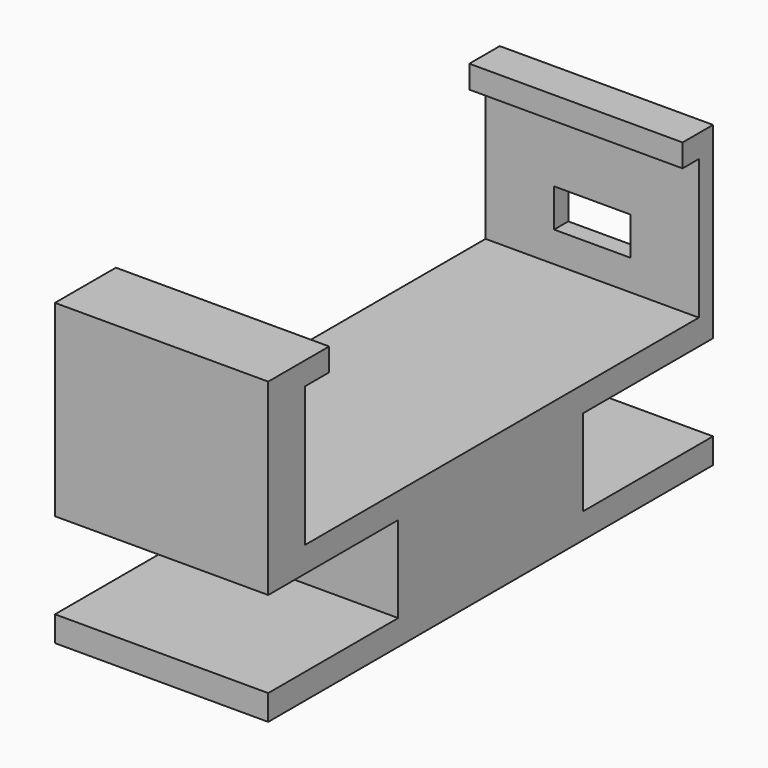
from build123d import *

# Parameters (mm, degrees)
F0_W      = 42
F0_H      = 109.5
F1_DEPTH  = 5
F2_W      = 42
F2_H      = 7.5
F2_H_2    = 15
F3_DEPTH  = 32
F4_W      = 42
F4_H      = 27.5
F5_DEPTH  = 4
F6_W      = 42
F6_H      = 27.5
F7_DEPTH  = 6
F8_W      = 15
F8_H      = 7.5
F9_DEPTH  = 3.501
F10_W     = 42
F10_H     = 54.75
F11_DEPTH = 22
F12_W     = 42
F12_H     = 17
F13_DEPTH = 32
F14_W     = 42
F14_H     = 17
F15_DEPTH = 32


# Not quite as in the source:
# - a feature names something its author has since deleted; it is built from what else it names


with BuildPart() as f1:
    # F0 (on Top) → F1 (new body)
    with BuildSketch(Plane.XY):
        Rectangle(F0_W, F0_H)
    extrude(amount=F1_DEPTH)

    # F2 (on face) → F3 (join)
    with BuildSketch(Plane.XY.offset(5)):
        with Locations((0, 51)):
            Rectangle(F2_W, F2_H)
        with Locations((0, -47.25)):
            Rectangle(F2_W, F2_H_2)
    extrude(amount=F3_DEPTH)

    # F4 (on face) → F5 (cut)
    with BuildSketch(Plane.XZ.offset(-47.25)):
        with Locations((0, 18.75)):
            Rectangle(F4_W, F4_H)
    extrude(amount=-F5_DEPTH, mode=Mode.SUBTRACT)

    # F6 (on face) → F7 (cut)
    with BuildSketch(Plane(origin=(0, -39.75, 0), x_dir=(-1, 0, 0), z_dir=(0, 1, 0))):
        with Locations((0, 18.75)):
            Rectangle(F6_W, F6_H)
    extrude(amount=-F7_DEPTH, mode=Mode.SUBTRACT)

    # F8 (on face) → F9 (cut, through all)
    with BuildSketch(Plane.XZ.offset(-51.25)):
        with Locations((0, 14.75)):
            Rectangle(F8_W, F8_H)
    extrude(amount=-F9_DEPTH, mode=Mode.SUBTRACT)

    # F10 (on face) → F11 (join)
    with BuildSketch(Plane(origin=(0, 0, 0), x_dir=(1, 0, 0), z_dir=(0, 0, -1))):
        with Locations((0, -27.375)):
            Rectangle(F10_W, F10_H)
        with Locations((0, 27.375)):
            Rectangle(F10_W, F10_H)
    extrude(amount=F11_DEPTH)

    # F12 (on face) → F13 (cut)
    with BuildSketch(Plane(origin=(0, 54.75, 0), x_dir=(-1, 0, 0), z_dir=(0, 1, 0))):
        with Locations((0, -8.5)):
            Rectangle(F12_W, F12_H)
    extrude(amount=-F13_DEPTH, mode=Mode.SUBTRACT)

    # F14 (on face) → F15 (cut)
    with BuildSketch(Plane.XZ.offset(54.75)):
        with Locations((0, -8.5)):
            Rectangle(F14_W, F14_H)
    extrude(amount=-F15_DEPTH, mode=Mode.SUBTRACT)


solid = f1.part
